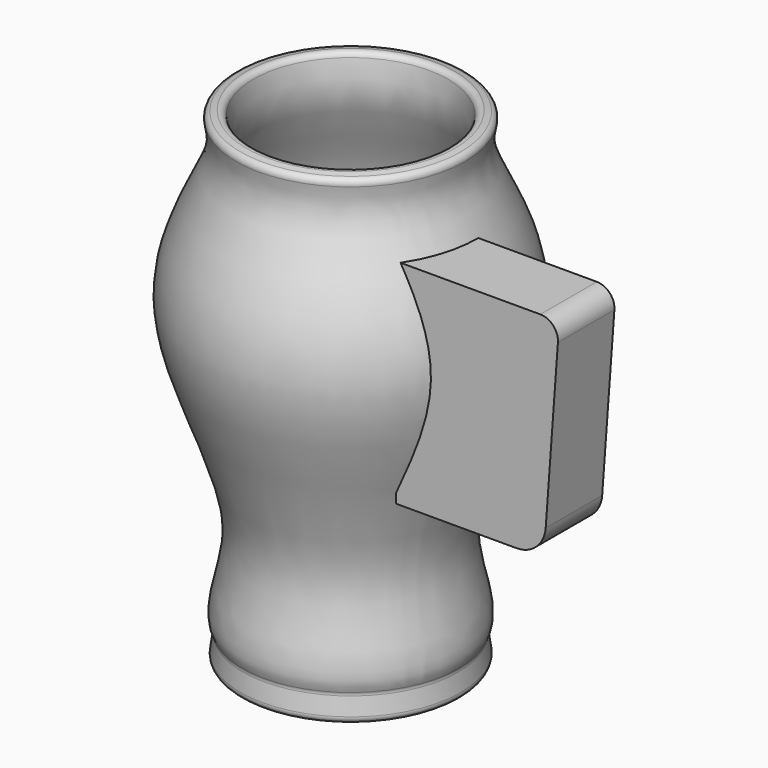
from build123d import *

# Parameters (mm, degrees)
F3_DEPTH = 12


# Not quite as in the source:
# - ends of sketch curves that miss each other by under 0.0002 mm in the source are joined
# - the dataset's text gives a spline's control points without its knots; the knots are read off the source's solid
# - a feature names something its author has since deleted; it is built from what else it names


with BuildPart() as f1:
    # F0 (on Front) → F1 (revolve)
    with BuildSketch(Plane.XZ):
        with BuildLine():
            Line((14, -34.9656030457), (0, -34.9656030457))
            Line((0, -34.9656030457), (0, -37.9656030457))
            Line((0, -37.9656030457), (13.0000005874, -37.9656030457))
            ThreePointArc((13.0000005874, -37.9656030457), (13.7071073686, -38.2584962646), (14.0000005874, -38.9656030457))
            Line((14.0000005874, -38.9656030457), (14.0000005874, -39.046891405))
            ThreePointArc((14.0000005874, -39.046891405), (14.2928938062, -39.7539981862), (15.0000005874, -40.046891405))
            Line((15.0000005874, -40.046891405), (17.7186424754, -40.046891405))
            ThreePointArc((17.7186424754, -40.046891405), (18.4738448885, -39.7023830643), (18.708700241, -38.9062300358))
            Line((18.708700241, -38.9062300358), (18.2957692257, -35.9997777484))
            ThreePointArc((18.2957692257, -35.9997777484), (18.2977444092, -35.7051916871), (18.3854701901, -35.4239639569))
            add(Edge.make_bspline(
                [(18.3854701901, -35.4239639569), (18.3938341208, -35.4066229273), (18.5266025306, -35.1277578366), (18.715877762, -34.5927520996), (18.9035078406, -33.6233183365), (18.9226821636, -32.5357112994), (18.7918928566, -31.3188454124), (18.5720759542, -30.1109709554), (18.2997668102, -28.8784920294), (18.0019168963, -27.6102199641), (17.7034756417, -26.3076373829), (17.4285036664, -24.9791398913), (17.2002452219, -23.6373442156), (17.0673042938, -22.5207488001), (17.0051081865, -21.6365836967), (16.9756231658, -20.7611172733), (16.9990707182, -19.6360514205), (17.1185949958, -18.2464350707), (17.3240335952, -16.8174640009), (17.7038966841, -14.8649802067), (18.3596277701, -12.3449239598), (19.3703268305, -9.2244095855), (20.9189772303, -4.9706404314), (22.6172956433, -0.6240335836), (24.1483643217, 3.7590439656), (25.1295783411, 7.0605692876), (25.7342965147, 9.8240580962), (26.0392862698, 12.0442976969), (26.1648967684, 13.7137703794), (26.1685337061, 15.3878187051), (26.0518454029, 17.0119822189), (25.8322638307, 18.5901337627), (25.4209698448, 20.627310439), (24.7216031829, 23.0459512807), (23.6964780756, 25.7409416359), (22.5885542227, 28.228790192), (21.4962267159, 30.5046914486), (20.6793388957, 32.21258168), (20.1289606437, 33.4488399425), (19.7787812598, 34.3036786221), (19.547325286, 34.9481723653), (19.4020021639, 35.416216841), (19.2833316507, 35.8518216962), (19.1727912273, 36.370793715), (19.0660440192, 37.1522073311), (19.0417766325, 38.0744005106), (19.1487238737, 39.1917477059), (19.3166912918, 40.104463848), (19.4330006188, 40.6519351293), (19.4594400571, 40.7741810345)],
                knots=[0.0463574991, 0.0463574991, 0.0463574991, 0.0463574991, 0.046875, 0.0546875, 0.0625, 0.078125, 0.09375, 0.109375, 0.125, 0.140625, 0.15625, 0.171875, 0.1875, 0.203125, 0.2109375, 0.21875, 0.234375, 0.25, 0.265625, 0.28125, 0.3125, 0.34375, 0.375, 0.4375, 0.46875, 0.5, 0.53125, 0.546875, 0.5625, 0.578125, 0.59375, 0.609375, 0.625, 0.65625, 0.6875, 0.71875, 0.75, 0.78125, 0.796875, 0.8125, 0.828125, 0.8359375, 0.84375, 0.859375, 0.875, 0.90625, 0.9375, 0.96875, 0.9775642332, 0.9775642332, 0.9775642332, 0.9775642332], degree=3))
            ThreePointArc((19.4594400571, 40.7741810345), (19.3241307475, 41.5246968677), (18.6990969993, 41.961608619))
            Line((18.6990969993, 41.961608619), (17.7229356258, 42.1787356599))
            ThreePointArc((17.7229356258, 42.1787356599), (16.9666270477, 42.04477858), (16.5284093417, 41.4139755943))
            add(Edge.make_bspline(
                [(14, -34.9656030457), (18.1488398757, -34.9656022334), (7.8272694156, -17.8536936323), (30.2740659447, 13.5701815718), (15.1317400386, 33.2891506405), (16.0855594241, 39.3663154938), (16.5284093417, 41.4139755943)],
                knots=[0, 0, 0, 0, 0.2139219808, 0.5688887366, 0.8382051703, 0.9776999292, 0.9776999292, 0.9776999292, 0.9776999292], degree=3))
        make_face()
    revolve(axis=Axis((0, 0, -36.4656030457), (0, 0, -1)))

    # F2 (on Front) → F3 (join)
    with BuildSketch(Plane.XZ):
        with BuildLine():
            Line((41.8363309535, 30.0700475706), (17.3273498321, 30.0700475706))
            Line((17.3273498321, 30.0700475706), (17.3273498321, -6.2283408547))
            Line((17.3273498321, -6.2283408547), (37.764269958, -6.2283408547))
            ThreePointArc((37.764269958, -6.2283408547), (41.1686061021, -4.8903751825), (42.7509882873, -1.592539022))
            Line((42.7509882873, -1.592539022), (44.828361951, 26.8515286702))
            ThreePointArc((44.828361951, 26.8515286702), (44.0335515502, 29.112649257), (41.8363309535, 30.0700475706))
        make_face()
    extrude(amount=F3_DEPTH)


solid = f1.part
